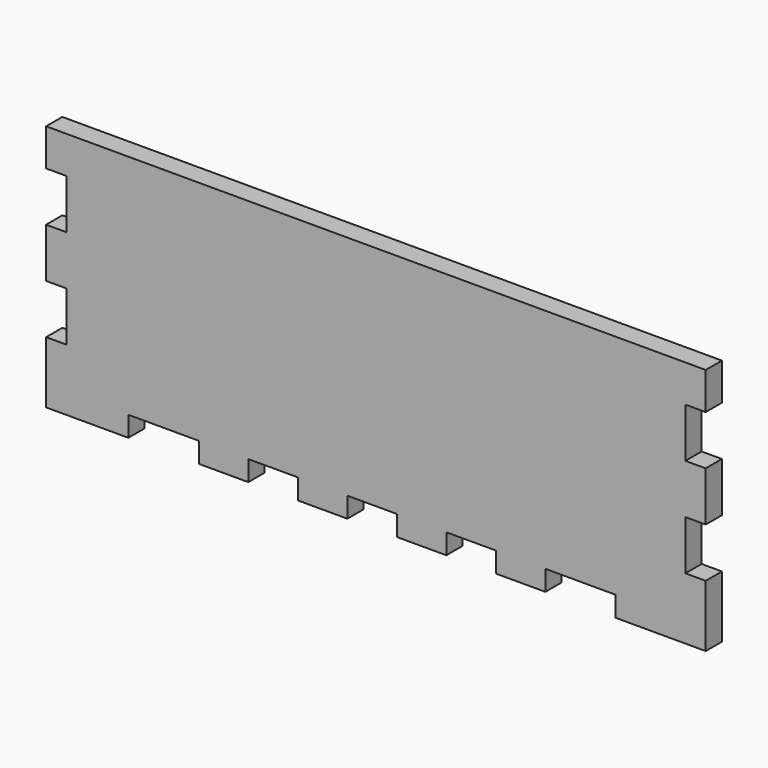
from build123d import *

# Parameters (mm, degrees)
F0_W     = 169.2275
F0_H     = 63.5
F1_DEPTH = 5.207
F2_W     = 5.207
F2_H     = 12.7
F2_W_2   = 12.7
F2_H_2   = 5.207
F2_W_3   = 18.097754
F3_DEPTH = 5.208


# Not quite as in the source:
# - a feature names something its author has since deleted; it is built from what else it names


with BuildPart() as f1:
    # F0 (on Front) → F1 (new body)
    with BuildSketch(Plane.XZ):
        Rectangle(F0_W, F0_H)
    extrude(amount=F1_DEPTH)

    # F2 (on face) → F3 (cut, through all)
    with BuildSketch(Plane(origin=(0, 0, 0), x_dir=(-1, 0, 0), z_dir=(0, 1, 0))):
        with Locations((-82.01025, 15.875)):
            Rectangle(F2_W, F2_H)
        with Locations((-82.01025, -9.525)):
            Rectangle(F2_W, F2_H)
        Polygon((-61.42101, -31.75), (-43.478704, -31.75), (-43.478704, -26.543), (-61.43371, -26.543), align=None)
        with Locations((-24.428704, -29.1465)):
            Rectangle(F2_W_2, F2_H_2)
        with Locations((0.971296, -29.1465)):
            Rectangle(F2_W_2, F2_H_2)
        with Locations((26.371296, -29.1465)):
            Rectangle(F2_W_2, F2_H_2)
        with Locations((54.470173, -29.1465)):
            Rectangle(F2_W_3, F2_H_2)
        with Locations((82.01025, 15.875)):
            Rectangle(F2_W, F2_H)
        with Locations((82.01025, -9.525)):
            Rectangle(F2_W, F2_H)
    extrude(amount=-F3_DEPTH, mode=Mode.SUBTRACT)


solid = f1.part
